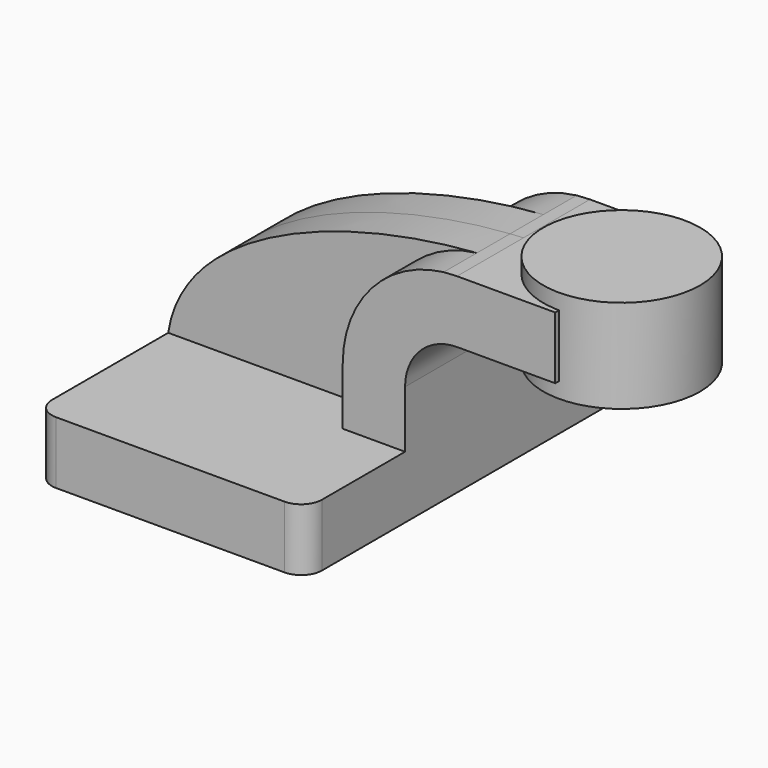
from build123d import *

# Parameters (mm, degrees)
F1_DEPTH = 63.5
F0_W     = 26.8478
F0_H     = 19.05
F2_DEPTH = 25.4
F3_DEPTH = 12.7
F5_R     = 6.35


# Not quite as in the source:
# - a feature names something its author has since deleted; it is built from what else it names


with BuildPart() as f1:
    # F0 (on Front) → F1 (new body, symmetric)
    with BuildSketch(Plane.XZ):
        Polygon((22.225, 9.525), (-41.275, 9.525), (-41.275, -9.525), (41.275, -9.525), (41.275, 9.525), align=None)
    extrude(amount=F1_DEPTH, both=True)

    # F0 (on Front) → F2 (join, symmetric)
    with BuildSketch(Plane.XZ):
        with BuildLine():
            Line((22.225, 27.0002), (22.225, 9.525))
            Line((22.225, 9.525), (41.275, 9.525))
            Line((41.275, 9.525), (41.275, 27.0002))
            ThreePointArc((41.275, 27.0002), (45.9246798487, 38.2255201513), (57.15, 42.8752))
            Line((57.15, 42.8752), (60.325, 42.8752))
            Line((60.325, 42.8752), (60.325, 61.9252))
            Line((60.325, 61.9252), (57.15, 61.9252))
            add(Edge.make_bspline(
                [(53.0632119302, 61.6852657816), (54.436822126, 61.7819257772), (55.7997974291, 61.8618933869), (57.15, 61.9252)],
                knots=[107.8202324218, 107.8202324218, 107.8202324218, 107.8202324218, 111.5045361635, 111.5045361635, 111.5045361635, 111.5045361635], degree=3))
            ThreePointArc((53.0632119302, 61.6852657816), (31.0493611349, 50.2060672717), (22.225, 27.0002))
        make_face()
        with Locations((73.7489, 52.4002)):
            Rectangle(F0_W, F0_H)
    extrude(amount=F2_DEPTH, both=True)

    # F0 (on Front) → F3 (join, symmetric)
    with BuildSketch(Plane.XZ):
        with BuildLine():
            add(Edge.make_bspline(
                [(-41.275, 9.525), (-36.4415043335, 41.7320166895), (12.8648512777, 58.8565350576), (53.0632119302, 61.6852657816)],
                knots=[0, 0, 0, 0, 107.8202324218, 107.8202324218, 107.8202324218, 107.8202324218], degree=3))
            Line((-41.275, 9.525), (22.225, 9.525))
            Line((22.225, 9.525), (22.225, 27.0002))
            ThreePointArc((22.225, 27.0002), (31.0493611349, 50.2060672717), (53.0632119302, 61.6852657816))
        make_face()
    extrude(amount=F3_DEPTH, both=True)

    # F5
    f5_edges = [f1.edges().sort_by_distance(p)[0] for p in [
        (-41.275, -63.5, 0),
        (41.275, -63.5, 0),
        (41.275, 63.5, 0),
        (-41.275, 63.5, 0),
    ]]
    fillet(f5_edges, radius=F5_R)


with BuildPart() as f4:
    # F0 (on Front) → F4 (revolve)
    with BuildSketch(Plane.XZ):
        Polygon((87.1728, 66.675), (87.1728, 61.9252), (87.1728, 42.8752), (87.1728, 38.1), (111.125, 38.1), (111.125, 66.675), align=None)
    revolve(axis=Axis((87.1728, 0, 52.3875), (0, 0, 1)))


solid = Compound([f1.part, f4.part])
